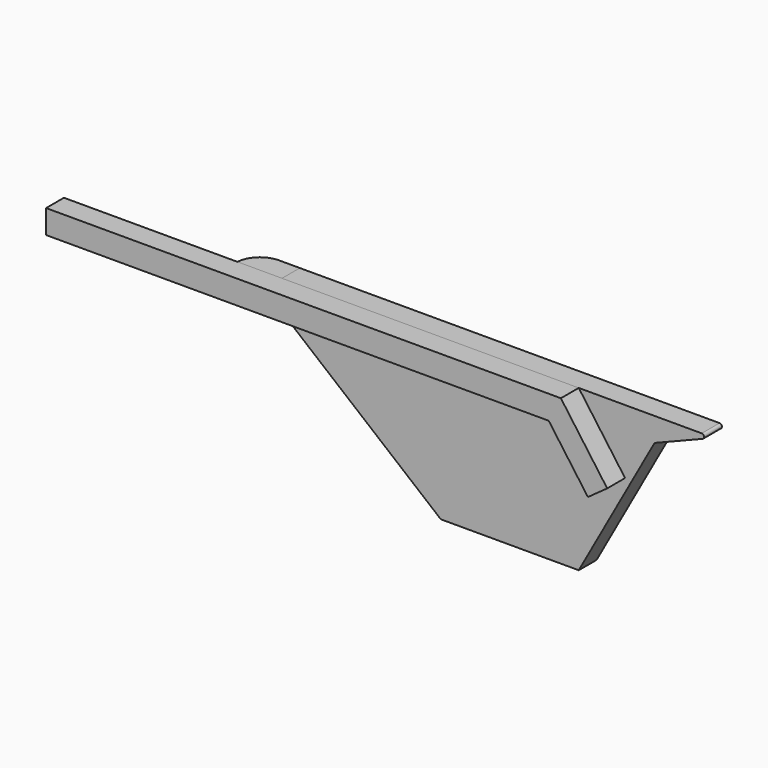
from build123d import *

# Parameters (mm, degrees)
F1_DEPTH    = 4.7625
F2_W        = 4.7625
F2_H        = 6.35
F3_DEPTH    = 9.525
F4_T1_DEPTH = 31.7003420835
F6_DEPTH    = 9.525
F8_DEPTH    = 4.7752


# Not quite as in the source:
# - a fillet or chamfer that OpenCascade refuses, or shapes differently, is made with other operations: its cross-section is extruded or revolved along the edge and cut away or added


with BuildPart() as f1:
    # F0 (on Front) → F1 (new body)
    with BuildSketch(Plane.XZ):
        with BuildLine():
            Line((-58.42, 0), (-28.9322432641, 0))
            Line((-28.9322432641, 0), (-12.7254, 29.2379192107))
            Line((-12.7254, 29.2379192107), (-2.4543888247, 33.3381232726))
            ThreePointArc((-2.4543888247, 33.3381232726), (-2.1438636322, 33.9058141101), (-2.6427305165, 34.3179192107))
            Line((-2.6427305165, 34.3179192107), (-12.7254, 34.3179192107))
            Line((-12.7254, 34.3179192107), (-28.8753250815, 34.3179192107))
            Line((-28.8753250815, 34.3179192107), (-92.3753250815, 34.3179192107))
            Line((-92.3753250815, 34.3179192107), (-92.3753250815, 27.9679192107))
            Line((-92.3753250815, 27.9679192107), (-58.42, 0))
        make_face()
    extrude(amount=F1_DEPTH)


with BuildPart() as f3:
    # F2 (on face) → F3 (new body)
    with BuildSketch(Plane(origin=(-92.3753250815, 0, 0), x_dir=(0, -1, 0), z_dir=(-1, 0, 0))):
        with Locations((2.38125, 31.1429192107)):
            Rectangle(F2_W, F2_H)
    extrude(amount=F3_DEPTH)

    # F4: fillet of radius 5.08 on 1 edges, made by hand

    # F4_s2 → F4_t1 (cut)
    with BuildSketch(Plane.XY.offset(15.2927481689)):
        with BuildLine():
            ThreePointArc((-96.8302566648, 0), (-100.308294905, -1.3773455468), (-101.9003250815, -4.7625))
            Line((-101.9003250815, -4.7625), (-101.9003250815, 0))
            Line((-101.9003250815, 0), (-96.8302566648, 0))
        make_face()
    extrude(amount=F4_T1_DEPTH, mode=Mode.SUBTRACT)


with BuildPart() as f6:
    # F5 (on face) → F6 (new body)
    with BuildSketch(Plane(origin=(0, 0, 0), x_dir=(-1, 0, 0), z_dir=(0, 1, 0))):
        with BuildLine():
            Line((54.0486851786, 25.4279192107), (54.0486851786, 18.2318821344))
            ThreePointArc((54.0486851786, 18.2318821344), (58.4936851786, 13.7868821344), (62.9386851786, 18.2318821344))
            Line((62.9386851786, 18.2318821344), (62.9386851786, 25.4279192107))
            Line((62.9386851786, 25.4279192107), (54.0486851786, 25.4279192107))
        make_face()
    extrude(amount=F6_DEPTH)


with BuildPart() as f8:
    # F7 (on face) → F8 (new body)
    with BuildSketch(Plane.XZ.offset(4.7625)):
        Polygon((-31.534574919, 29.2379192107), (-28.9322432641, 25.6231317048), (-28.9322432641, 34.3179192107), (-138.9904432641, 34.3179192107), (-138.9904432641, 29.2379192107), (-35.3291034698, 29.2379192107), align=None)
        Polygon((-28.9322432641, 34.3179192107), (-28.9322432641, 25.6231317048), (-23.1566244349, 17.6004668216), (-19.0338594402, 20.5684979532), align=None)
    extrude(amount=F8_DEPTH)


solid = Compound([f1.part, f3.part, f6.part, f8.part])
